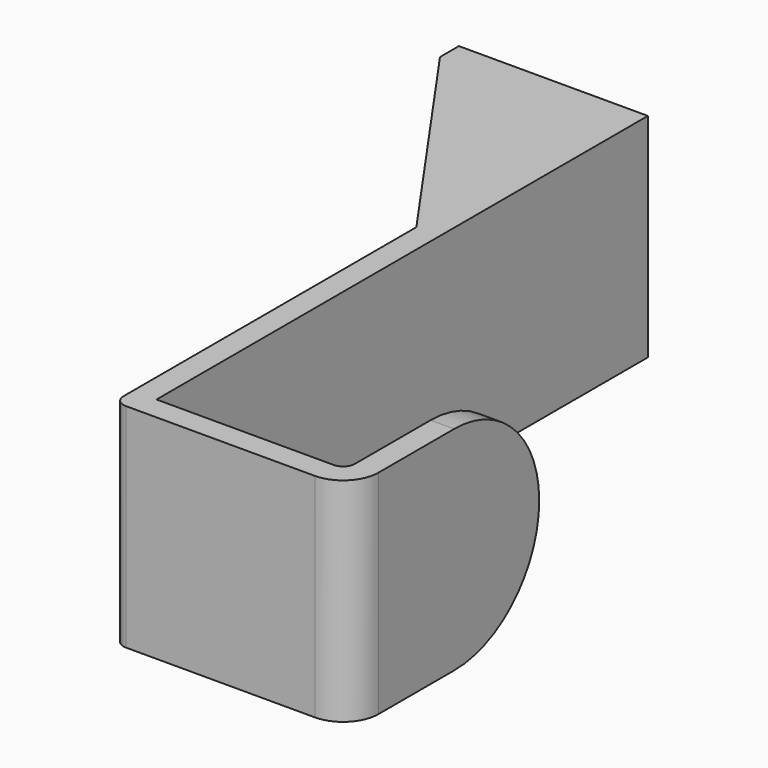
from build123d import *

# Parameters (mm, degrees)
F0_W     = 2
F0_H     = 18
F1_DEPTH = 18
F2_R     = 1
F3_DEPTH = 25
F4_R     = 3
F5_R     = 1
F6_R     = 1
F7_R     = 8.99999


# Not quite as in the source:
# - a fillet or chamfer is up to 0.001 mm smaller than in the source, because OpenCascade refuses the exact size


with BuildPart() as f1:
    # F0 (on Top) → F1 (new body)
    with BuildSketch(Plane.XY):
        Polygon((-1, 5), (-1, -25), (1, -25), (1, 25), (-1, 25), align=None)
        Polygon((1, -25), (-1, -25), (-1, -27), (19, -27), (19, -25), (17, -25), align=None)
        Polygon((-15, 25), (-1, 5), (-1, 25), align=None)
        Polygon((-1, 25), (1, 25), (1, 27), (-15, 27), (-15, 25), align=None)
        with Locations((18, -16)):
            Rectangle(F0_W, F0_H)
    extrude(amount=F1_DEPTH)

    # F2 (on face) → F3 (cut)
    with BuildSketch(Plane(origin=(0, 27, 0), x_dir=(-1, 0, 0), z_dir=(0, 1, 0))):
        with Locations((9, 9)):
            Circle(F2_R)
        with Locations((13, 9)):
            Circle(F2_R)
    extrude(amount=-F3_DEPTH, mode=Mode.SUBTRACT)

    # F4
    f4_edges = [f1.edges().sort_by_distance(p)[0] for p in [
        (19, -27, 9),
    ]]
    fillet(f4_edges, radius=F4_R)

    # F5
    f5_edges = [f1.edges().sort_by_distance(p)[0] for p in [
        (17, -25, 9),
    ]]
    fillet(f5_edges, radius=F5_R)

    # F6
    f6_edges = [f1.edges().sort_by_distance(p)[0] for p in [
        (-1, -27, 9),
    ]]
    fillet(f6_edges, radius=F6_R)

    # F7 (radius 9 in the source; OpenCascade refuses exactly that, so slightly less here)
    f7_edges = [f1.edges().sort_by_distance(p)[0] for p in [
        (18, -7, 18),
        (18, -7, 0),
    ]]
    fillet(f7_edges, radius=F7_R)


solid = f1.part
